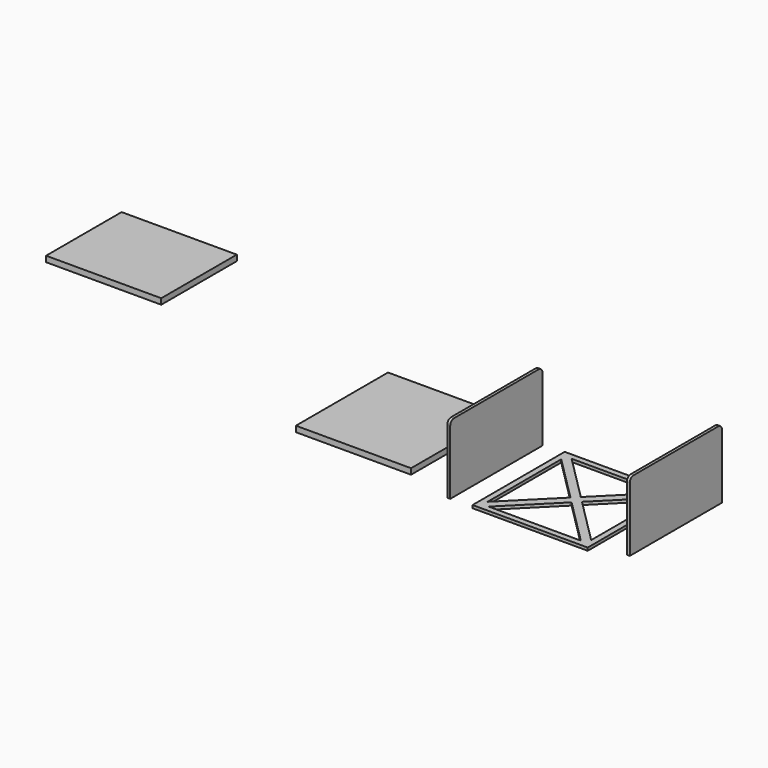
from build123d import *

# Parameters (mm, degrees)
F0_W      = 6.35
F0_H      = 6.35
F1_DEPTH  = 3.175
F2_W      = 3.175
F2_H      = 127
F3_DEPTH  = 76.2
F4_W      = 3.175
F4_H      = 127
F5_DEPTH  = 76.2
F6_W      = 127
F6_H      = 127
F7_DEPTH  = 6.35
F8_R      = 5.08
F9_R      = 5.08
F10_R     = 5.08
F11_R     = 5.08
F12_W     = 127
F12_H     = 104.14
F13_DEPTH = 6.35


# Not quite as in the source:
# - a length typed as a fraction of an inch, garbled in the dataset ("3 / 203.2 mm" for 3/8 in), is restored


with BuildPart() as f1:
    # F0 (on Top) → F1 (new body)
    with BuildSketch(Plane.XY):
        Polygon((-34.5571719459, -84.5880480751), (-40.9071719459, -84.5880480751), (-40.9071719459, -90.9380480751), (86.0928280541, -90.9380480751), (86.0928280541, -84.5880480751), (79.7428280541, -84.5880480751), (73.3928280541, -84.5880480751), (63.2345444911, -84.5880480751), (-28.2071719459, -84.5880480751), align=None)
        Polygon((79.7428280541, -78.2380480751), (28.9428280541, -27.4380480751), (22.5928280541, -33.7880480751), (73.3928280541, -84.5880480751), (73.3928280541, -78.2380480751), align=None)
        with Locations((76.5678280541, -81.4130480751)):
            Rectangle(F0_W, F0_H)
        with Locations((-31.3821719459, -81.4130480751)):
            Rectangle(F0_W, F0_H)
        Polygon((16.2428280541, -27.4380480751), (-34.5571719459, -78.2380480751), (-28.2071719459, -78.2380480751), (-28.2071719459, -84.5880480751), (22.5928280541, -33.7880480751), align=None)
        Polygon((22.5928280541, -21.0880480751), (-28.2071719459, 29.7119519249), (-28.2071719459, 23.3619519249), (-34.5498589529, 23.3619519249), (-34.5498505211, 23.3546305002), (16.2428280541, -27.4380480751), align=None)
        Polygon((28.9428280541, -27.4380480751), (22.5928280541, -21.0880480751), (16.2428280541, -27.4380480751), (22.5928280541, -33.7880480751), align=None)
        Polygon((73.3928280541, 23.3619519249), (73.3928280541, 29.7119519249), (22.5928280541, -21.0880480751), (28.9428280541, -27.4380480751), (79.7428280541, 23.3619519249), align=None)
        with Locations((76.5678280541, 26.5369519249)):
            Rectangle(F0_W, F0_H)
        Polygon((-28.2071719459, 29.7119519249), (-34.5571719459, 29.7119519249), (-34.5498589529, 23.3619519249), (-28.2071719459, 23.3619519249), align=None)
        Polygon((-40.9071719459, 29.7119519249), (-34.5571719459, 29.7119519249), (-28.2071719459, 29.7119519249), (73.3928280541, 29.7119519249), (79.7428280541, 29.7119519249), (86.0928280541, 29.7119519249), (86.0928280541, 36.0619519249), (-40.9071719459, 36.0619519249), align=None)
        Polygon((-34.5571719459, 23.3619519249), (-34.5571719459, 29.7119519249), (-40.9071719459, 29.7119519249), (-40.9071719459, -84.5880480751), (-34.5571719459, -84.5880480751), (-34.5571719459, -78.2380480751), align=None)
        Polygon((86.0928280541, 29.7119519249), (79.7428280541, 29.7119519249), (79.7428280541, 23.3619519249), (79.7428280541, -78.2380480751), (79.7428280541, -84.5880480751), (86.0928280541, -84.5880480751), align=None)
    extrude(amount=F1_DEPTH)


with BuildPart() as f3:
    # F2 (on Top) → F3 (new body)
    with BuildSketch(Plane.XY):
        with Locations((-68.4703838587, -25.738487184)):
            Rectangle(F2_W, F2_H)
    extrude(amount=F3_DEPTH)

    # F8
    f8_edges = [f3.edges().sort_by_distance(p)[0] for p in [
        (-68.470384, -89.238487, 76.2),
    ]]
    fillet(f8_edges, radius=F8_R)

    # F9
    f9_edges = [f3.edges().sort_by_distance(p)[0] for p in [
        (-68.470384, 37.761513, 76.2),
    ]]
    fillet(f9_edges, radius=F9_R)


with BuildPart() as f5:
    # F4 (on Top) → F5 (new body)
    with BuildSketch(Plane.XY):
        with Locations((118.7510346651, -12.2532194257)):
            Rectangle(F4_W, F4_H)
    extrude(amount=F5_DEPTH)

    # F10
    f10_edges = [f5.edges().sort_by_distance(p)[0] for p in [
        (118.751035, -75.753219, 76.2),
    ]]
    fillet(f10_edges, radius=F10_R)

    # F11
    f11_edges = [f5.edges().sort_by_distance(p)[0] for p in [
        (118.751035, 51.246781, 76.2),
    ]]
    fillet(f11_edges, radius=F11_R)


with BuildPart() as f7:
    # F6 (on Top) → F7 (new body)
    with BuildSketch(Plane.XY):
        with Locations((-192.4403140545, -2.1958520412)):
            Rectangle(F6_W, F6_H)
    extrude(amount=-F7_DEPTH)


with BuildPart() as f13:
    # F12 (on Top) → F13 (new body)
    with BuildSketch(Plane.XY):
        with Locations((-550.8351667404, 90.0116942596)):
            Rectangle(F12_W, F12_H)
    extrude(amount=F13_DEPTH)


solid = Compound([f1.part, f3.part, f5.part, f7.part, f13.part])
